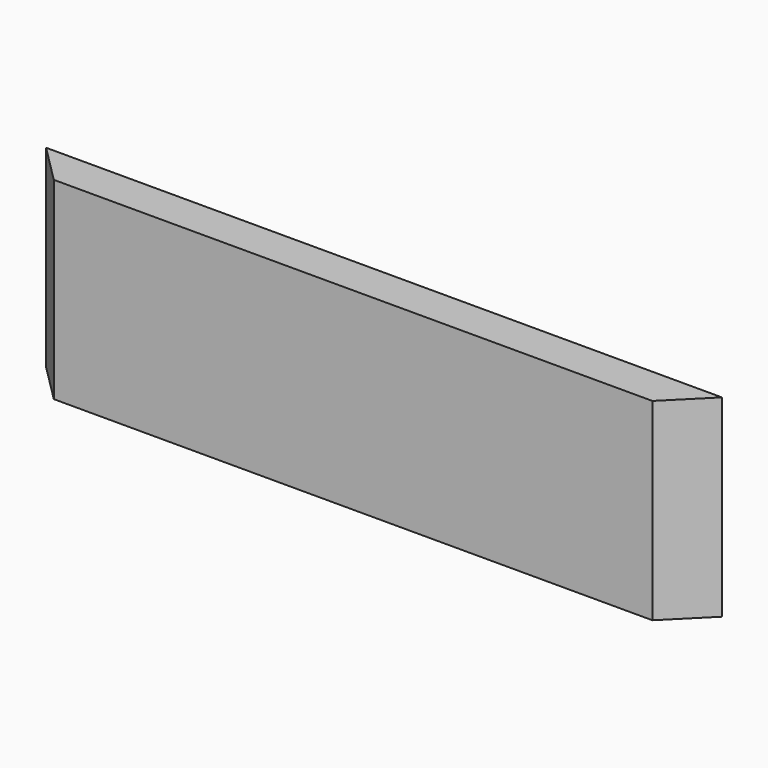
from build123d import *

# Parameters (mm, degrees)
F0_W     = 350
F0_H     = 100
F1_DEPTH = 10
F2_SIZE2 = 19.99999
F2_SIZE  = 19.99999
F3_SIZE2 = 19.99999
F3_SIZE  = 19.99999


# Not quite as in the source:
# - a fillet or chamfer is up to 0.001 mm smaller than in the source, because OpenCascade refuses the exact size


with BuildPart() as f1:
    # F0 (on Front) → F1 (new body, symmetric)
    with BuildSketch(Plane.XZ):
        with Locations((175, 50)):
            Rectangle(F0_W, F0_H)
    extrude(amount=F1_DEPTH, both=True)

    # F2 (size 20 and 20 in the source; OpenCascade refuses exactly that, so slightly less here)
    f2_edges = [f1.edges().sort_by_distance(p)[0] for p in [
        (0, -10, 50),
    ]]
    chamfer(f2_edges, length=F2_SIZE, length2=F2_SIZE2)

    # F3 (size 20 and 20 in the source; OpenCascade refuses exactly that, so slightly less here)
    f3_edges = [f1.edges().sort_by_distance(p)[0] for p in [
        (350, -10, 50),
    ]]
    chamfer(f3_edges, length=F3_SIZE, length2=F3_SIZE2)


solid = f1.part
